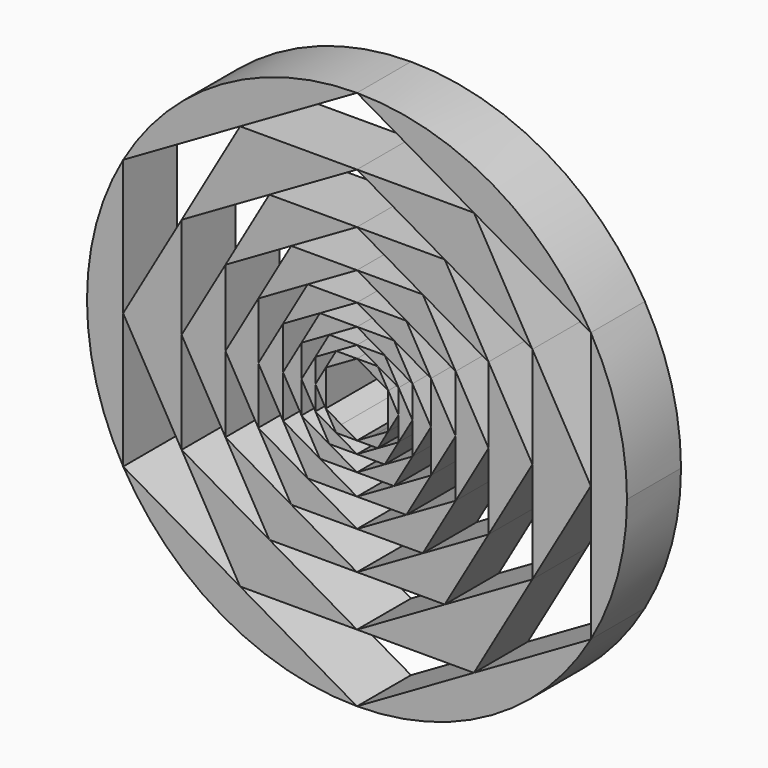
from build123d import *

# Parameters (mm, degrees)
F1_DEPTH = 25.4


with BuildPart() as f1:
    # F0 (on Front) → F1 (new body)
    with BuildSketch(Plane.XZ):
        with BuildLine():
            ThreePointArc((87.9881810245, -50.8), (98.138063951, -26.2960149824), (101.6, 0))
            ThreePointArc((101.6, 0), (98.138063951, 26.2960149824), (87.9881810245, 50.8))
            Line((87.9881810245, 50.8), (87.9881810245, 0))
            Line((87.9881810245, 0), (87.9881810245, -50.8))
        make_face()
    extrude(amount=F1_DEPTH)


with BuildPart() as f1b:
    # F0 (on Front) → F1, piece 2 (new body)
    with BuildSketch(Plane.XZ):
        with BuildLine():
            Line((43.9940905122, 76.2), (87.9881810245, 50.8))
            ThreePointArc((87.9881810245, 50.8), (50.8, 87.9881810245), (0, 101.6))
            Line((0, 101.6), (43.9940905122, 76.2))
        make_face()
    extrude(amount=F1_DEPTH)


with BuildPart() as f1c:
    # F0 (on Front) → F1, piece 3 (new body)
    with BuildSketch(Plane.XZ):
        with BuildLine():
            ThreePointArc((0, -101.6), (50.8, -87.9881810245), (87.9881810245, -50.8))
            Line((87.9881810245, -50.8), (43.9940905122, -76.2))
            Line((43.9940905122, -76.2), (0, -101.6))
        make_face()
    extrude(amount=F1_DEPTH)


with BuildPart() as f1d:
    # F0 (on Front) → F1, piece 4 (new body)
    with BuildSketch(Plane.XZ):
        with BuildLine():
            Line((-43.9940905122, 76.2), (0, 101.6))
            ThreePointArc((0, 101.6), (-50.8, 87.9881810245), (-87.9881810245, 50.8))
            Line((-87.9881810245, 50.8), (-43.9940905122, 76.2))
        make_face()
    extrude(amount=F1_DEPTH)


with BuildPart() as f1e:
    # F0 (on Front) → F1, piece 5 (new body)
    with BuildSketch(Plane.XZ):
        Polygon((65.9911357684, 38.1), (43.9940905122, 76.2), (0, 76.2), (32.9955678842, 57.15), align=None)
    extrude(amount=F1_DEPTH)


with BuildPart() as f1f:
    # F0 (on Front) → F1, piece 6 (new body)
    with BuildSketch(Plane.XZ):
        Polygon((65.9911357684, -38.1), (87.9881810245, 0), (65.9911357684, 38.1), (65.9911357684, 0), align=None)
    extrude(amount=F1_DEPTH)


with BuildPart() as f1g:
    # F0 (on Front) → F1, piece 7 (new body)
    with BuildSketch(Plane.XZ):
        with BuildLine():
            ThreePointArc((-87.9881810245, -50.8), (-50.8, -87.9881810245), (0, -101.6))
            Line((0, -101.6), (-43.9940905122, -76.2))
            Line((-43.9940905122, -76.2), (-87.9881810245, -50.8))
        make_face()
    extrude(amount=F1_DEPTH)


with BuildPart() as f1h:
    # F0 (on Front) → F1, piece 8 (new body)
    with BuildSketch(Plane.XZ):
        Polygon((0, -76.2), (43.9940905122, -76.2), (65.9911357684, -38.1), (32.9955678842, -57.15), align=None)
    extrude(amount=F1_DEPTH)


with BuildPart() as f1i:
    # F0 (on Front) → F1, piece 9 (new body)
    with BuildSketch(Plane.XZ):
        with BuildLine():
            Line((-87.9881810245, 0), (-87.9881810245, 50.8))
            ThreePointArc((-87.9881810245, 50.8), (-101.6, 0), (-87.9881810245, -50.8))
            Line((-87.9881810245, -50.8), (-87.9881810245, 0))
        make_face()
    extrude(amount=F1_DEPTH)


with BuildPart() as f1j:
    # F0 (on Front) → F1, piece 10 (new body)
    with BuildSketch(Plane.XZ):
        Polygon((0, 76.2), (-43.9940905122, 76.2), (-65.9911357684, 38.1), (-32.9955678842, 57.15), align=None)
    extrude(amount=F1_DEPTH)


with BuildPart() as f1k:
    # F0 (on Front) → F1, piece 11 (new body)
    with BuildSketch(Plane.XZ):
        Polygon((-65.9911357684, -38.1), (-43.9940905122, -76.2), (0, -76.2), (-32.9955678842, -57.15), align=None)
    extrude(amount=F1_DEPTH)


with BuildPart() as f1l:
    # F0 (on Front) → F1, piece 12 (new body)
    with BuildSketch(Plane.XZ):
        Polygon((-65.9911357684, 38.1), (-87.9881810245, 0), (-65.9911357684, -38.1), (-65.9911357684, 0), align=None)
    extrude(amount=F1_DEPTH)


with BuildPart() as f1m:
    # F0 (on Front) → F1, piece 13 (new body)
    with BuildSketch(Plane.XZ):
        Polygon((49.4933518263, 28.575), (32.9955678842, 57.15), (0, 57.15), (24.7466759131, 42.8625), align=None)
    extrude(amount=F1_DEPTH)


with BuildPart() as f1n:
    # F0 (on Front) → F1, piece 14 (new body)
    with BuildSketch(Plane.XZ):
        Polygon((0, 57.15), (-32.9955678842, 57.15), (-49.4933518263, 28.575), (-24.7466759131, 42.8625), align=None)
    extrude(amount=F1_DEPTH)


with BuildPart() as f1o:
    # F0 (on Front) → F1, piece 15 (new body)
    with BuildSketch(Plane.XZ):
        Polygon((49.4933518263, -28.575), (65.9911357684, 0), (49.4933518263, 28.575), (49.4933518263, 0), align=None)
    extrude(amount=F1_DEPTH)


with BuildPart() as f1p:
    # F0 (on Front) → F1, piece 16 (new body)
    with BuildSketch(Plane.XZ):
        Polygon((0, -57.15), (32.9955678842, -57.15), (49.4933518263, -28.575), (24.7466759131, -42.8625), align=None)
    extrude(amount=F1_DEPTH)


with BuildPart() as f1q:
    # F0 (on Front) → F1, piece 17 (new body)
    with BuildSketch(Plane.XZ):
        Polygon((-49.4933518263, -28.575), (-32.9955678842, -57.15), (0, -57.15), (-24.7466759131, -42.8625), align=None)
    extrude(amount=F1_DEPTH)


with BuildPart() as f1r:
    # F0 (on Front) → F1, piece 18 (new body)
    with BuildSketch(Plane.XZ):
        Polygon((-49.4933518263, 28.575), (-65.9911357684, 0), (-49.4933518263, -28.575), (-49.4933518263, 0), align=None)
    extrude(amount=F1_DEPTH)


with BuildPart() as f1s:
    # F0 (on Front) → F1, piece 19 (new body)
    with BuildSketch(Plane.XZ):
        Polygon((37.1200138697, 21.43125), (24.7466759131, 42.8625), (0, 42.8625), (18.5600069349, 32.146875), align=None)
    extrude(amount=F1_DEPTH)


with BuildPart() as f1t:
    # F0 (on Front) → F1, piece 20 (new body)
    with BuildSketch(Plane.XZ):
        Polygon((0, 42.8625), (-24.7466759131, 42.8625), (-37.1200138697, 21.43125), (-18.5600069349, 32.146875), align=None)
    extrude(amount=F1_DEPTH)


with BuildPart() as f1u:
    # F0 (on Front) → F1, piece 21 (new body)
    with BuildSketch(Plane.XZ):
        Polygon((37.1200138697, -21.43125), (49.4933518263, 0), (37.1200138697, 21.43125), (37.1200138697, 0), align=None)
    extrude(amount=F1_DEPTH)


with BuildPart() as f1v:
    # F0 (on Front) → F1, piece 22 (new body)
    with BuildSketch(Plane.XZ):
        Polygon((-37.1200138697, 21.43125), (-49.4933518263, 0), (-37.1200138697, -21.43125), (-37.1200138697, 0), align=None)
    extrude(amount=F1_DEPTH)


with BuildPart() as f1w:
    # F0 (on Front) → F1, piece 23 (new body)
    with BuildSketch(Plane.XZ):
        Polygon((0, -42.8625), (24.7466759131, -42.8625), (37.1200138697, -21.43125), (18.5600069349, -32.146875), align=None)
    extrude(amount=F1_DEPTH)


with BuildPart() as f1x:
    # F0 (on Front) → F1, piece 24 (new body)
    with BuildSketch(Plane.XZ):
        Polygon((-37.1200138697, -21.43125), (-24.7466759131, -42.8625), (0, -42.8625), (-18.5600069349, -32.146875), align=None)
    extrude(amount=F1_DEPTH)


with BuildPart() as f1y:
    # F0 (on Front) → F1, piece 25 (new body)
    with BuildSketch(Plane.XZ):
        Polygon((27.8400104023, 16.0734375), (18.5600069349, 32.146875), (0, 32.146875), (13.9200052011, 24.11015625), align=None)
    extrude(amount=F1_DEPTH)


with BuildPart() as f1z:
    # F0 (on Front) → F1, piece 26 (new body)
    with BuildSketch(Plane.XZ):
        Polygon((0, 32.146875), (-18.5600069349, 32.146875), (-27.8400104023, 16.0734375), (-13.9200052011, 24.11015625), align=None)
    extrude(amount=F1_DEPTH)


with BuildPart() as f1ba:
    # F0 (on Front) → F1, piece 27 (new body)
    with BuildSketch(Plane.XZ):
        Polygon((27.8400104023, -16.0734375), (37.1200138697, 0), (27.8400104023, 16.0734375), (27.8400104023, 0), align=None)
    extrude(amount=F1_DEPTH)


with BuildPart() as f1bb:
    # F0 (on Front) → F1, piece 28 (new body)
    with BuildSketch(Plane.XZ):
        Polygon((-27.8400104023, 16.0734375), (-37.1200138697, 0), (-27.8400104023, -16.0734375), (-27.8400104023, 0), align=None)
    extrude(amount=F1_DEPTH)


with BuildPart() as f1bc:
    # F0 (on Front) → F1, piece 29 (new body)
    with BuildSketch(Plane.XZ):
        Polygon((0, -32.146875), (18.5600069349, -32.146875), (27.8400104023, -16.0734375), (13.9200052011, -24.11015625), align=None)
    extrude(amount=F1_DEPTH)


with BuildPart() as f1bd:
    # F0 (on Front) → F1, piece 30 (new body)
    with BuildSketch(Plane.XZ):
        Polygon((-27.8400104023, -16.0734375), (-18.5600069349, -32.146875), (0, -32.146875), (-13.9200052011, -24.11015625), align=None)
    extrude(amount=F1_DEPTH)


with BuildPart() as f1be:
    # F0 (on Front) → F1, piece 31 (new body)
    with BuildSketch(Plane.XZ):
        Polygon((20.8800078017, 12.055078125), (13.9200052011, 24.11015625), (0, 24.11015625), (10.4400039009, 18.0826171875), align=None)
    extrude(amount=F1_DEPTH)


with BuildPart() as f1bf:
    # F0 (on Front) → F1, piece 32 (new body)
    with BuildSketch(Plane.XZ):
        Polygon((0, 24.11015625), (-13.9200052011, 24.11015625), (-20.8800078017, 12.055078125), (-10.4400039009, 18.0826171875), align=None)
    extrude(amount=F1_DEPTH)


with BuildPart() as f1bg:
    # F0 (on Front) → F1, piece 33 (new body)
    with BuildSketch(Plane.XZ):
        Polygon((20.8800078017, -12.055078125), (27.8400104023, 0), (20.8800078017, 12.055078125), (20.8800078017, 0), align=None)
    extrude(amount=F1_DEPTH)


with BuildPart() as f1bh:
    # F0 (on Front) → F1, piece 34 (new body)
    with BuildSketch(Plane.XZ):
        Polygon((-20.8800078017, 12.055078125), (-27.8400104023, 0), (-20.8800078017, -12.055078125), (-20.8800078017, 0), align=None)
    extrude(amount=F1_DEPTH)


with BuildPart() as f1bi:
    # F0 (on Front) → F1, piece 35 (new body)
    with BuildSketch(Plane.XZ):
        Polygon((0, -24.11015625), (13.9200052011, -24.11015625), (20.8800078017, -12.055078125), (10.4400039009, -18.0826171875), align=None)
    extrude(amount=F1_DEPTH)


with BuildPart() as f1bj:
    # F0 (on Front) → F1, piece 36 (new body)
    with BuildSketch(Plane.XZ):
        Polygon((-20.8800078017, -12.055078125), (-13.9200052011, -24.11015625), (0, -24.11015625), (-10.4400039009, -18.0826171875), align=None)
    extrude(amount=F1_DEPTH)


with BuildPart() as f1bk:
    # F0 (on Front) → F1, piece 37 (new body)
    with BuildSketch(Plane.XZ):
        Polygon((15.6600058513, 9.0413085938), (10.4400039009, 18.0826171875), (0, 18.0826171875), (7.8300029256, 13.5619628906), align=None)
    extrude(amount=F1_DEPTH)


with BuildPart() as f1bl:
    # F0 (on Front) → F1, piece 38 (new body)
    with BuildSketch(Plane.XZ):
        Polygon((0, 18.0826171875), (-10.4400039009, 18.0826171875), (-15.6600058513, 9.0413085937), (-7.8300029256, 13.5619628906), align=None)
    extrude(amount=F1_DEPTH)


with BuildPart() as f1bm:
    # F0 (on Front) → F1, piece 39 (new body)
    with BuildSketch(Plane.XZ):
        Polygon((15.6600058513, -9.0413085937), (20.8800078017, 0), (15.6600058513, 9.0413085938), (15.6600058513, 0), align=None)
    extrude(amount=F1_DEPTH)


with BuildPart() as f1bn:
    # F0 (on Front) → F1, piece 40 (new body)
    with BuildSketch(Plane.XZ):
        Polygon((-15.6600058513, 9.0413085937), (-20.8800078017, 0), (-15.6600058513, -9.0413085938), (-15.6600058513, 0), align=None)
    extrude(amount=F1_DEPTH)


with BuildPart() as f1bo:
    # F0 (on Front) → F1, piece 41 (new body)
    with BuildSketch(Plane.XZ):
        Polygon((0, -18.0826171875), (10.4400039009, -18.0826171875), (15.6600058513, -9.0413085937), (7.8300029256, -13.5619628906), align=None)
    extrude(amount=F1_DEPTH)


with BuildPart() as f1bp:
    # F0 (on Front) → F1, piece 42 (new body)
    with BuildSketch(Plane.XZ):
        Polygon((-15.6600058513, -9.0413085938), (-10.4400039009, -18.0826171875), (0, -18.0826171875), (-7.8300029256, -13.5619628906), align=None)
    extrude(amount=F1_DEPTH)


with BuildPart() as f1bq:
    # F0 (on Front) → F1, piece 43 (new body)
    with BuildSketch(Plane.XZ):
        Polygon((11.7450043885, 6.7809814453), (7.8300029256, 13.5619628906), (0, 13.5619628906), (5.8725021942, 10.171472168), align=None)
    extrude(amount=F1_DEPTH)


with BuildPart() as f1br:
    # F0 (on Front) → F1, piece 44 (new body)
    with BuildSketch(Plane.XZ):
        Polygon((0, 13.5619628906), (-7.8300029256, 13.5619628906), (-11.7450043885, 6.7809814453), (-5.8725021942, 10.171472168), align=None)
    extrude(amount=F1_DEPTH)


with BuildPart() as f1bs:
    # F0 (on Front) → F1, piece 45 (new body)
    with BuildSketch(Plane.XZ):
        Polygon((11.7450043885, -6.7809814453), (15.6600058513, 0), (11.7450043885, 6.7809814453), (11.7450043885, 0), align=None)
    extrude(amount=F1_DEPTH)


with BuildPart() as f1bt:
    # F0 (on Front) → F1, piece 46 (new body)
    with BuildSketch(Plane.XZ):
        Polygon((-11.7450043885, 6.7809814453), (-15.6600058513, 0), (-11.7450043885, -6.7809814453), (-11.7450043885, 0), align=None)
    extrude(amount=F1_DEPTH)


with BuildPart() as f1bu:
    # F0 (on Front) → F1, piece 47 (new body)
    with BuildSketch(Plane.XZ):
        Polygon((0, -13.5619628906), (7.8300029256, -13.5619628906), (11.7450043885, -6.7809814453), (5.8725021942, -10.171472168), align=None)
    extrude(amount=F1_DEPTH)


with BuildPart() as f1bv:
    # F0 (on Front) → F1, piece 48 (new body)
    with BuildSketch(Plane.XZ):
        Polygon((-11.7450043885, -6.7809814453), (-7.8300029256, -13.5619628906), (0, -13.5619628906), (-5.8725021942, -10.171472168), align=None)
    extrude(amount=F1_DEPTH)


solid = Compound([f1.part, f1b.part, f1c.part, f1d.part, f1e.part, f1f.part, f1g.part, f1h.part, f1i.part, f1j.part, f1k.part, f1l.part, f1m.part, f1n.part, f1o.part, f1p.part, f1q.part, f1r.part, f1s.part, f1t.part, f1u.part, f1v.part, f1w.part, f1x.part, f1y.part, f1z.part, f1ba.part, f1bb.part, f1bc.part, f1bd.part, f1be.part, f1bf.part, f1bg.part, f1bh.part, f1bi.part, f1bj.part, f1bk.part, f1bl.part, f1bm.part, f1bn.part, f1bo.part, f1bp.part, f1bq.part, f1br.part, f1bs.part, f1bt.part, f1bu.part, f1bv.part])
